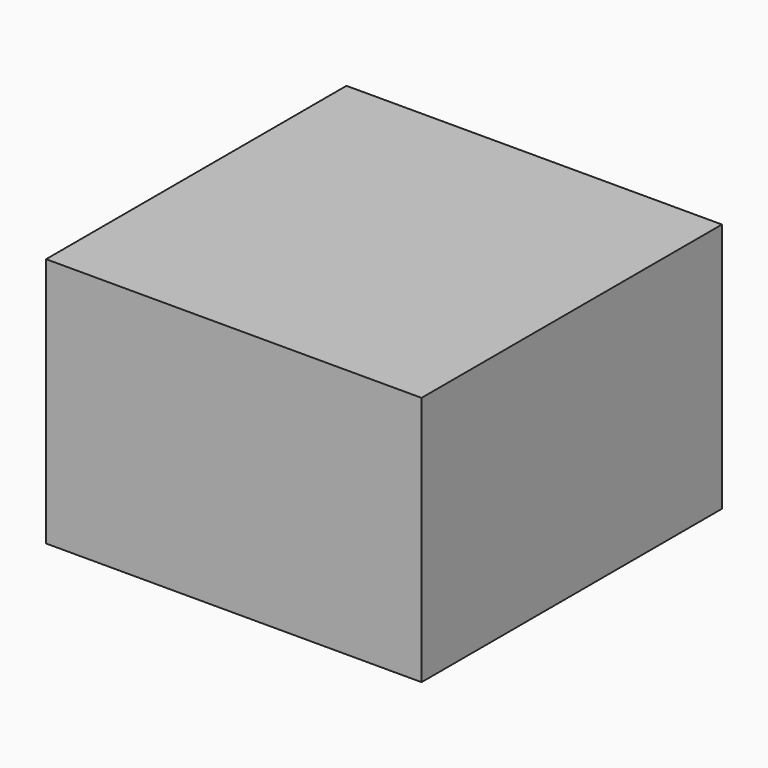
from build123d import *

# Parameters (mm, degrees)
F0_W     = 76.2
F0_H     = 76.2
F1_DEPTH = 50.8


# Not quite as in the source:
# - the program builds the solid bodies; features that only make, move or delete a surface that nothing else refers to are left out


with BuildPart() as f1:
    # F0 (on Top) → F1 (new body)
    with BuildSketch(Plane.XY):
        Rectangle(F0_W, F0_H)
    extrude(amount=F1_DEPTH)


solid = f1.part
